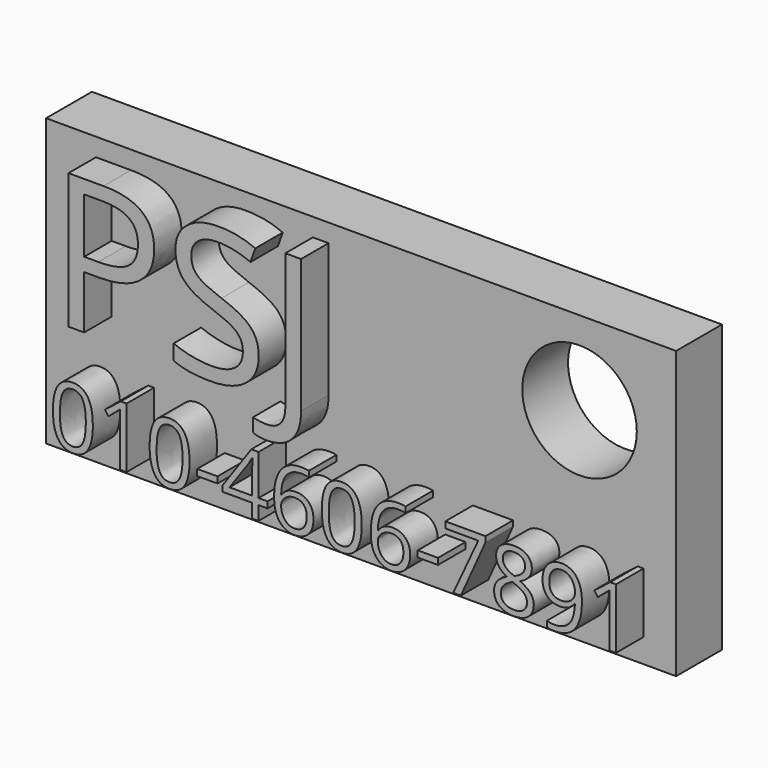
from build123d import *

# Parameters (mm, degrees)
F0_W           = 55
F0_H           = 25
F1_DEPTH       = 5
F2_TEXT_SIZE   = 16.5281832472
F2_TEXT_SIZE_2 = 7.38058445
F3_DEPTH       = 3
F4_R           = 5
F5_DEPTH       = 5.001


# Not quite as in the source:
# - Text() gives the source's letters only with a copy of the font that has no kerning and outlines rounded to 1/6400 em; it was checked with that copy


with BuildPart() as f1:
    # F0 (on Front) → F1 (new body)
    with BuildSketch(Plane.XZ):
        with Locations((27.5, 12.5)):
            Rectangle(F0_W, F0_H)
    extrude(amount=F1_DEPTH)

    # F2 (on face) → F3 (join)
    with BuildSketch(Plane.XZ.offset(5)):
        with Locations((2.7328250905, 11.6157410995)):
            Text('PSJ', F2_TEXT_SIZE, font='Open Sans', text_align=(TextAlign.LEFT, TextAlign.BOTTOM))
        with Locations((2.6310570538, 2.0866936538)):
            Text('010-4606-7891', F2_TEXT_SIZE_2, font='Open Sans', text_align=(TextAlign.LEFT, TextAlign.BOTTOM))
    extrude(amount=F3_DEPTH)

    # F4 (on face) → F5 (cut, through all)
    with BuildSketch(Plane.XZ.offset(5)):
        with Locations((46.5689448228, 17.6915321499)):
            Circle(F4_R)
    extrude(amount=-F5_DEPTH, mode=Mode.SUBTRACT)


solid = f1.part
